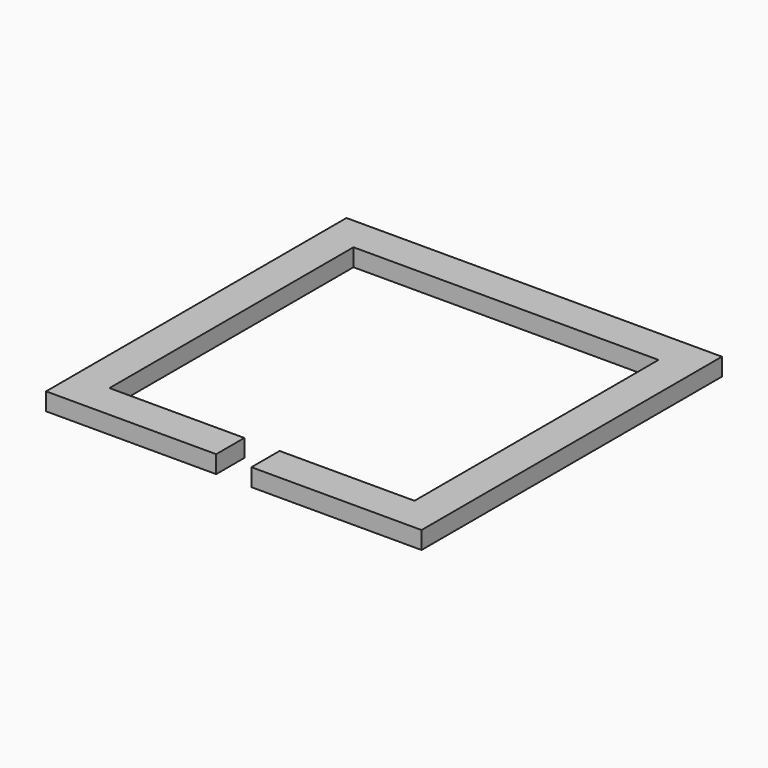
from build123d import *

# Parameters (mm, degrees)
F1_DEPTH = 3.175


# Not quite as in the source:
# - a length typed as a fraction of an inch, garbled in the dataset ("3 / 203.2 mm" for 3/8 in), is restored


with BuildPart() as f1:
    # F0 (on Top) → F1 (new body)
    with BuildSketch(Plane.XY):
        Polygon((33.85, 0), (-33.85, 0), (-33.85, -67.7), (-3.175, -67.7), (-3.175, -61.35), (-27.5, -61.35), (-27.5, -6.35), (27.5, -6.35), (27.5, -61.35), (3.175, -61.35), (3.175, -67.7), (33.85, -67.7), align=None)
    extrude(amount=F1_DEPTH)


solid = f1.part
